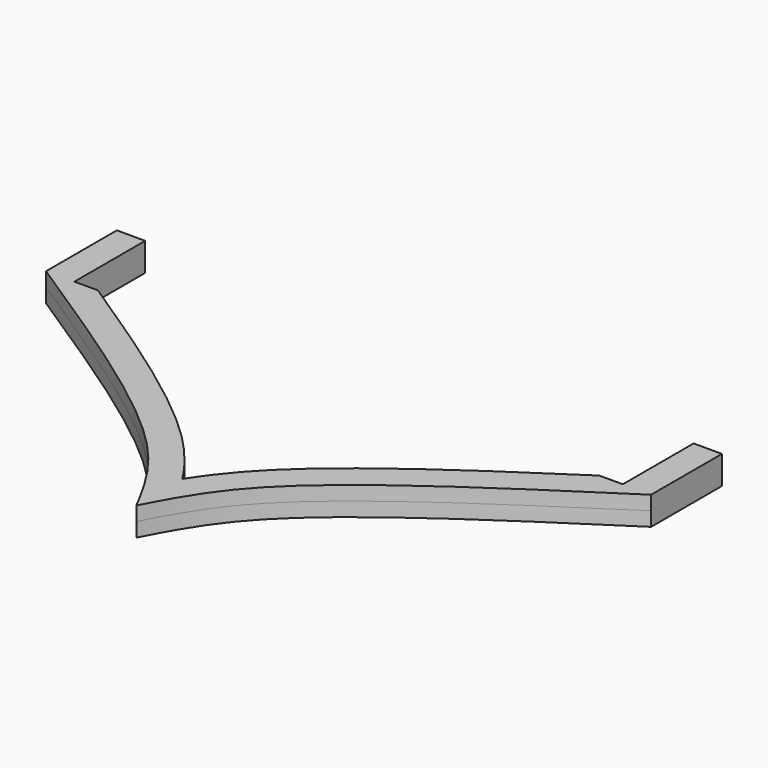
from build123d import *

# Parameters (mm, degrees)
F1_DEPTH = 1.6


# Not quite as in the source:
# - ends of sketch curves that miss each other by under 0.0002 mm in the source are joined
# - the dataset's text gives a spline's control points without its knots; the knots are read off the source's solid


with BuildPart() as f1:
    # F0 (on Top) → F1 (new body, symmetric)
    with BuildSketch(Plane.XY):
        with BuildLine():
            Line((-34.2, 10), (-34.2, 0))
            add(Edge.make_bspline(
                [(-34.2, 0), (-23.4194875058, -7.0082505667), (-6.1932623577, -18.2067629029), (-1.6863845234, -26.7887792616), (0, -30)],
                knots=[0, 0, 0, 0, 0.6258197836, 1, 1, 1, 1], degree=3))
            add(Edge.make_bspline(
                [(34.2, 0), (23.4194875058, -7.0082505667), (6.1932623577, -18.2067629029), (1.6863845234, -26.7887792616), (0, -30)],
                knots=[0, 0, 0, 0, 0.6258197836, 1, 1, 1, 1], degree=3))
            Line((34.2, 0), (34.2, 10))
            Line((34.2, 10), (31, 10))
            Line((31, 10), (31, -1.5827e-06))
            Line((31, -1.5827e-06), (28.3359270428, -2.9003e-06))
            add(Edge.make_bspline(
                [(28.3359270428, -2.9003e-06), (27.5607449913, -0.5065418318), (24.6516596419, -2.413093867), (19.716056361, -5.7054487071), (14.8542229798, -9.1340817117), (11.2931387966, -11.828618628), (8.8128396772, -13.8240729179), (6.9255024837, -15.4669040903), (5.5358836916, -16.7716059599), (4.5551898562, -17.7483300719), (3.6448796139, -18.7193799543), (2.527802473, -19.9972589807), (1.2959036926, -21.5670975587), (0.4338110826, -22.8265648279), (0.0236068363, -23.4640566667), (2.5351e-06, -23.5008747441)],
                knots=[0.0798000576, 0.0798000576, 0.0798000576, 0.0798000576, 0.125, 0.25, 0.375, 0.4375, 0.5, 0.5625, 0.59375, 0.625, 0.65625, 0.6875, 0.75, 0.8125, 0.8163350073, 0.8163350073, 0.8163350073, 0.8163350073], degree=3))
            add(Edge.make_bspline(
                [(-28.335925148, -6e-10), (-27.5607449913, -0.5065418318), (-24.6516596419, -2.413093867), (-19.716056361, -5.7054487071), (-14.8542229798, -9.1340817117), (-11.2931387966, -11.828618628), (-8.8128396772, -13.8240729179), (-6.9255024837, -15.4669040903), (-5.5358836916, -16.7716059599), (-4.5551898562, -17.7483300719), (-3.6448796139, -18.7193799543), (-2.527802473, -19.9972589807), (-1.2959036926, -21.5670975587), (-0.4338110826, -22.8265648279), (-0.0236068363, -23.4640566667), (2.5351e-06, -23.5008747441)],
                knots=[0.0798000576, 0.0798000576, 0.0798000576, 0.0798000576, 0.125, 0.25, 0.375, 0.4375, 0.5, 0.5625, 0.59375, 0.625, 0.65625, 0.6875, 0.75, 0.8125, 0.8163350073, 0.8163350073, 0.8163350073, 0.8163350073], degree=3))
            Line((-28.335925148, -6e-10), (-31, -1.5827e-06))
            Line((-31, -1.5827e-06), (-31, 10))
            Line((-31, 10), (-34.2, 10))
        make_face()
    extrude(amount=F1_DEPTH, both=True)


solid = f1.part
